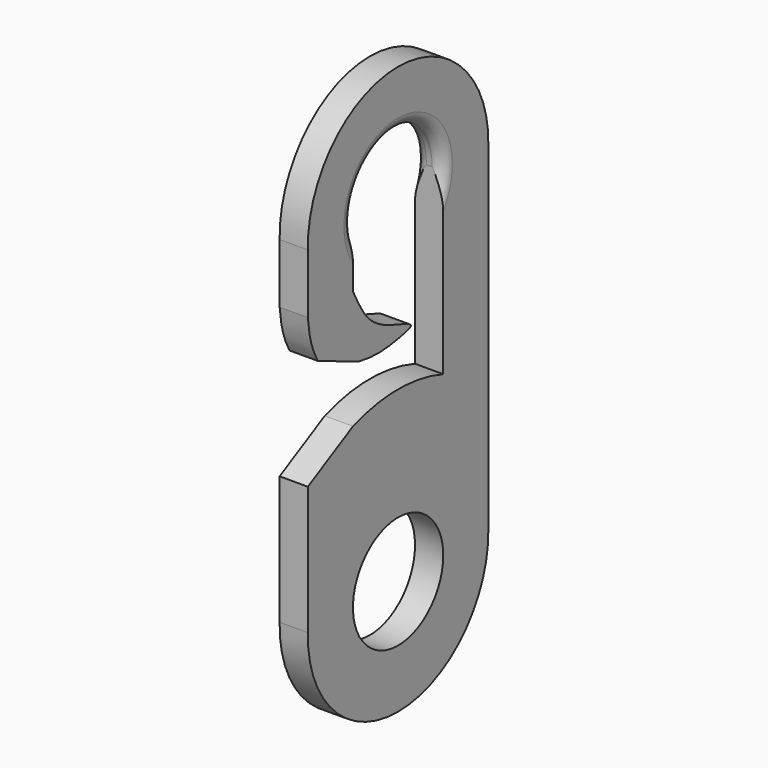
from build123d import *

# Parameters (mm, degrees)
F0_R        = 6.35
F1_DEPTH    = 3.175
F2_T1_DEPTH = 3.2744561413
F2_T4_ANGLE = 281.2740332969
F2_T6_ANGLE = 281.2740332969


# Not quite as in the source:
# - a fillet or chamfer that OpenCascade refuses, or shapes differently, is made with other operations: its cross-section is extruded or revolved along the edge and cut away or added


with BuildPart() as f1:
    # F0 (on Right) → F1 (new body)
    with BuildSketch(Plane.YZ):
        with BuildLine():
            Line((6.35, 19.05), (6.35, -1.0894877579))
            ThreePointArc((6.35, -1.0894877579), (0, 0), (-6.35, -1.0894877579))
            add(Edge.make_bspline(
                [(-6.35, -1.0894877579), (-8.4666666667, -2.2262237484), (-10.5833333333, -3.3629597389), (-12.7, -4.4996957295)],
                knots=[0, 0, 0, 0, 7.2077748584, 7.2077748584, 7.2077748584, 7.2077748584], degree=3))
            Line((-12.7, -4.4996957295), (-12.7, -18.9636734782))
            ThreePointArc((-12.7, -18.9636734782), (0, -31.9618793041), (12.7, -18.9636734782))
            Line((12.7, -18.9636734782), (12.7, 18.9636734782))
            ThreePointArc((12.7, 18.9636734782), (0, 31.9618793041), (-12.7, 18.9636734782))
            Line((-12.7, 18.9636734782), (-12.7, 12.2655965388))
            add(Edge.make_bspline(
                [(-12.7, 12.2655965388), (-12.5460680886, 10.8009133444), (-12.3921361771, 9.3362301501), (-11.3107701764, 7.4001117609)],
                knots=[0, 0, 0, 0, 0.2800418332, 0.2800418332, 0.2800418332, 0.2800418332], degree=3))
            add(Edge.make_bspline(
                [(-5.5794117662, 5), (-7.4898645696, 5.8000372536), (-9.400317373, 6.6000745073), (-11.3107701764, 7.4001117609)],
                knots=[0, 0, 0, 0, 6.2136145432, 6.2136145432, 6.2136145432, 6.2136145432], degree=3))
            add(Edge.make_bspline(
                [(-5.5794117662, 5), (-5.5956610435, 6.8858619014), (-5.9728305218, 9.5757292201), (-6.35, 12.2655965388)],
                knots=[0.7796078974, 0.7796078974, 0.7796078974, 0.7796078974, 1, 1, 1, 1], degree=3))
            Line((-6.35, 12.2655965388), (-6.35, 19.05))
            ThreePointArc((-6.35, 19.05), (0, 25.6118793041), (6.35, 19.05))
        make_face()
        with Locations((0, -19.05)):
            Circle(F0_R, mode=Mode.SUBTRACT)
        with BuildLine():
            add(Edge.make_bspline(
                [(-5.5794117662, 5), (-3.2248544463, 4.5091538123), (-0.6564824192, 4.8391769932), (3.3416252338, 5.6570567656), (-3.834716226, 7.1463236629), (-5.3129484548, 10.1981831131), (-6.35, 12.2655965388)],
                knots=[0, 0, 0, 0, 0.2814277691, 0.4456370567, 0.7068849416, 1, 1, 1, 1], degree=3))
            add(Edge.make_bspline(
                [(-5.5794117662, 5), (-5.5956610435, 6.8858619014), (-5.9728305218, 9.5757292201), (-6.35, 12.2655965388)],
                knots=[0.7796078974, 0.7796078974, 0.7796078974, 0.7796078974, 1, 1, 1, 1], degree=3))
        make_face()
    extrude(amount=F1_DEPTH)

    # F2: fillet of radius 1.27 on 4 edges, made by hand

    # F2_s2 → F2_t1 (cut)
    with BuildSketch(Plane.YZ.offset(-0.0497280707)):
        with BuildLine():
            ThreePointArc((-6.3505698659, 19.0681499948), (-6.3501424745, 19.0491315173), (-6.35, 19.0301087717))
            Line((-6.35, 19.0301087717), (-6.35, 19.05))
            ThreePointArc((-6.35, 19.05), (-6.3502914173, 19.0590747938), (-6.3505698659, 19.0681499948))
        make_face()
        with BuildLine():
            ThreePointArc((6.3505698659, 19.0681499948), (6.3501424745, 19.0491315173), (6.35, 19.0301087717))
            Line((6.35, 19.0301087717), (6.35, 19.05))
            ThreePointArc((6.35, 19.05), (6.3502914173, 19.0590747938), (6.3505698659, 19.0681499948))
        make_face()
    extrude(amount=F2_T1_DEPTH, mode=Mode.SUBTRACT)

    # F2_s3 → F2_t4 (revolve, cut)
    with BuildSketch(Plane(origin=(0, -9.4434175303, 7.7466985416), x_dir=(1, 0, 0), z_dir=(0, 0.7731434877, -0.6342311467))):
        with BuildLine():
            ThreePointArc((1.27, -8.5361310993), (0.3719743879, -8.1641567114), (0, -7.2661310993))
            Line((0, -7.2661310993), (0, -8.5361310993))
            Line((0, -8.5361310993), (1.27, -8.5361310993))
        make_face()
    revolve(axis=Axis((0, 0, 19.2584585737), (-1, 0, 0)), revolution_arc=F2_T4_ANGLE, mode=Mode.SUBTRACT)

    # F2_s5 → F2_t6 (revolve, cut)
    with BuildSketch(Plane(origin=(0, -9.4434175303, 7.7466985416), x_dir=(1, 0, 0), z_dir=(0, 0.7731434877, -0.6342311467))):
        with BuildLine():
            ThreePointArc((1.905, -8.5361310993), (2.8030256121, -8.1641567114), (3.175, -7.2661310993))
            Line((3.175, -7.2661310993), (3.175, -8.5361310993))
            Line((3.175, -8.5361310993), (1.905, -8.5361310993))
        make_face()
    revolve(axis=Axis((3.175, 0, 19.2584585737), (-1, 0, 0)), revolution_arc=F2_T6_ANGLE, mode=Mode.SUBTRACT)


solid = f1.part
